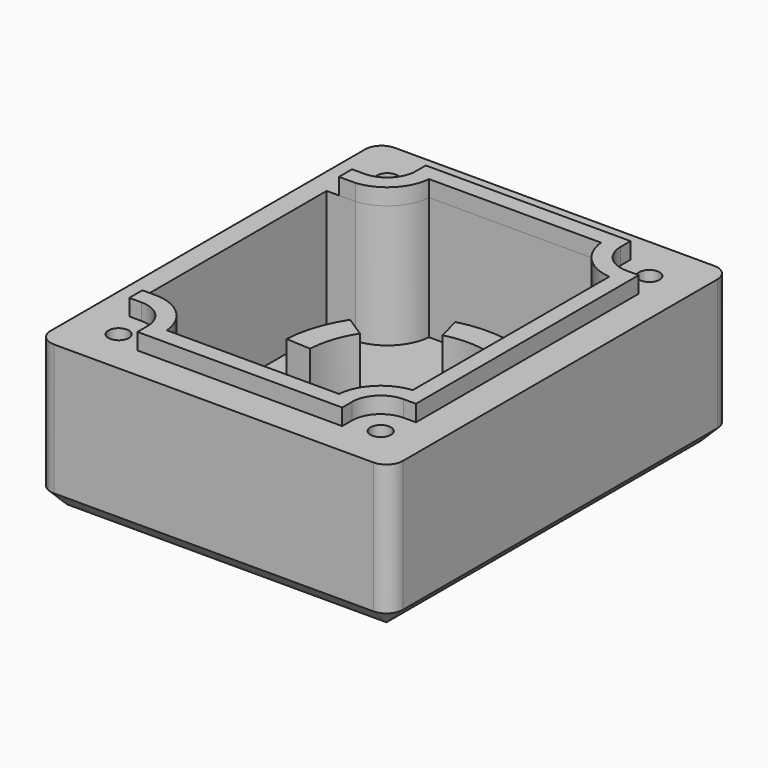
from build123d import *

# Parameters (mm, degrees)
F2_DEPTH  = 2
F3_DEPTH  = 3
F4_R      = 4.5
F5_DEPTH  = 5
F7_D      = 2.5
F8_R      = 4.5
F9_DEPTH  = 2
F10_DEPTH = 10
F11_DEPTH = 5
F12_DEPTH = 5
F13_R     = 4.5
F14_DEPTH = 15
F16_DEPTH = 7
F18_COUNT = 5
F19_SIZE  = 1.99999


# Not quite as in the source:
# - a fillet or chamfer is up to 0.001 mm smaller than in the source, because OpenCascade refuses the exact size


with BuildPart() as f2:
    # F1 (on Top) → F2 (new body)
    with BuildSketch(Plane.XY):
        with BuildLine():
            Line((-15.14, 17), (-16.64, 17))
            Line((-16.64, 17), (-16.64, -17))
            Line((-16.64, -17), (-15.14, -17))
            ThreePointArc((-15.14, -17), (-12.6651262658, -18.0251262658), (-11.64, -20.5))
            Line((-11.64, -20.5), (-11.64, -22))
            Line((-11.64, -22), (13.36, -22))
            Line((13.36, -22), (13.36, -20.5))
            ThreePointArc((13.36, -20.5), (14.3851262658, -18.0251262658), (16.86, -17))
            Line((16.86, -17), (18.36, -17))
            Line((18.36, -17), (18.36, 17))
            Line((18.36, 17), (16.86, 17))
            ThreePointArc((16.86, 17), (14.3851262658, 18.0251262658), (13.36, 20.5))
            Line((13.36, 20.5), (13.36, 22))
            Line((13.36, 22), (-11.64, 22))
            Line((-11.64, 22), (-11.64, 20.5))
            ThreePointArc((-11.64, 20.5), (-12.6651262658, 18.0251262658), (-15.14, 17))
        make_face()
    extrude(amount=F2_DEPTH)

    # F0 (on Top) → F3 (join)
    with BuildSketch(Plane.XY):
        with BuildLine():
            Line((20.36, 26), (-18.64, 26))
            ThreePointArc((-18.64, 26), (-20.0542135624, 25.4142135624), (-20.64, 24))
            Line((-20.64, 24), (-20.64, -24))
            ThreePointArc((-20.64, -24), (-20.0542135624, -25.4142135624), (-18.64, -26))
            Line((-18.64, -26), (20.36, -26))
            ThreePointArc((20.36, -26), (21.7742135624, -25.4142135624), (22.36, -24))
            Line((22.36, -24), (22.36, 24))
            ThreePointArc((22.36, 24), (21.7742135624, 25.4142135624), (20.36, 26))
        make_face()
        with BuildLine():
            Line((-17.64, -18), (-17.64, 18))
            Line((-17.64, 18), (-15.14, 18))
            ThreePointArc((-15.14, 18), (-13.372233047, 18.732233047), (-12.64, 20.5))
            Line((-12.64, 20.5), (-12.64, 23))
            Line((-12.64, 23), (14.36, 23))
            Line((14.36, 23), (14.36, 20.5))
            ThreePointArc((14.36, 20.5), (15.092233047, 18.732233047), (16.86, 18))
            Line((16.86, 18), (19.36, 18))
            Line((19.36, 18), (19.36, -18))
            Line((19.36, -18), (16.86, -18))
            ThreePointArc((16.86, -18), (15.092233047, -18.732233047), (14.36, -20.5))
            Line((14.36, -20.5), (14.36, -23))
            Line((14.36, -23), (-12.64, -23))
            Line((-12.64, -23), (-12.64, -20.5))
            ThreePointArc((-12.64, -20.5), (-13.372233047, -18.732233047), (-15.14, -18))
            Line((-15.14, -18), (-17.64, -18))
        make_face(mode=Mode.SUBTRACT)
        with BuildLine():
            Line((-15.14, 18), (-17.64, 18))
            Line((-17.64, 18), (-17.64, -18))
            Line((-17.64, -18), (-15.14, -18))
            ThreePointArc((-15.14, -18), (-13.372233047, -18.732233047), (-12.64, -20.5))
            Line((-12.64, -20.5), (-12.64, -23))
            Line((-12.64, -23), (14.36, -23))
            Line((14.36, -23), (14.36, -20.5))
            ThreePointArc((14.36, -20.5), (15.092233047, -18.732233047), (16.86, -18))
            Line((16.86, -18), (19.36, -18))
            Line((19.36, -18), (19.36, 18))
            Line((19.36, 18), (16.86, 18))
            ThreePointArc((16.86, 18), (15.092233047, 18.732233047), (14.36, 20.5))
            Line((14.36, 20.5), (14.36, 23))
            Line((14.36, 23), (-12.64, 23))
            Line((-12.64, 23), (-12.64, 20.5))
            ThreePointArc((-12.64, 20.5), (-13.372233047, 18.732233047), (-15.14, 18))
        make_face()
    extrude(amount=-F3_DEPTH)

    # F4 (on face) → F5 (cut, through all)
    with BuildSketch(Plane(origin=(0, 0, -3), x_dir=(1, 0, 0), z_dir=(0, 0, -1))):
        with Locations((2.36, 0)):
            Circle(F4_R)
    extrude(amount=-F5_DEPTH, mode=Mode.SUBTRACT)

    # F7 (through all)
    with Locations(Plane(origin=(0, 0, -3), x_dir=(1, 0, 0), z_dir=(0, 0, -1))):
        with Locations((-15.14, 20.5), (16.86, 20.5), (16.86, -20.5), (-15.14, -20.5)):
            Hole(F7_D / 2)

    # F8 (on face) → F9 (cut, through all)
    with BuildSketch(Plane.XY.offset(2)):
        with BuildLine():
            Line((11.36, 20), (-9.64, 20))
            ThreePointArc((-9.64, 20), (-11.234875162, 16.594875162), (-14.64, 15))
            Line((-14.64, 15), (-16.64, 15))
            Line((-16.64, 15), (-16.64, -15))
            Line((-16.64, -15), (-14.64, -15))
            ThreePointArc((-14.64, -15), (-11.234875162, -16.594875162), (-9.64, -20))
            Line((-9.64, -20), (11.36, -20))
            ThreePointArc((11.36, -20), (12.954875162, -16.594875162), (16.36, -15))
            Line((16.36, -15), (16.36, 15))
            ThreePointArc((16.36, 15), (12.954875162, 16.594875162), (11.36, 20))
        make_face()
        with Locations((2.36, 0)):
            Circle(F8_R, mode=Mode.SUBTRACT)
    extrude(amount=-F9_DEPTH, mode=Mode.SUBTRACT)

    # F10 (add): a face of the model
    f10_faces = [f2.faces().sort_by_distance(p)[0] for p in [
        (0.86, 25.3252407837, -3),
    ]]
    extrude(f10_faces, amount=F10_DEPTH)

    # F11 (add): a face of the model
    f11_faces = [f2.faces().sort_by_distance(p)[0] for p in [
        (0.86, 25.3252407837, 0),
    ]]
    extrude(f11_faces, amount=F11_DEPTH)

    # F12 (add): a face of the model
    f12_faces = [f2.faces().sort_by_distance(p)[0] for p in [
        (12.7977722881, -21.25, 2),
    ]]
    extrude(f12_faces, amount=F12_DEPTH)

    # F13 (on face) → F14 (cut)
    with BuildSketch(Plane.XY.offset(5)):
        with BuildLine():
            Line((-18.14, -15), (-16.64, -15))
            Line((-16.64, -15), (-14.64, -15))
            ThreePointArc((-14.64, -15), (-11.234875162, -16.594875162), (-9.64, -20))
            Line((-9.64, -20), (11.36, -20))
            ThreePointArc((11.36, -20), (12.954875162, -16.594875162), (16.36, -15))
            Line((16.36, -15), (16.36, 15))
            ThreePointArc((16.36, 15), (12.954875162, 16.594875162), (11.36, 20))
            Line((11.36, 20), (-9.64, 20))
            ThreePointArc((-9.64, 20), (-11.234875162, 16.594875162), (-14.64, 15))
            Line((-14.64, 15), (-16.64, 15))
            Line((-16.64, 15), (-18.14, 15))
            Line((-18.14, 15), (-18.14, -15))
        make_face()
        with Locations((2.36, 0)):
            Circle(F13_R, mode=Mode.SUBTRACT)
    extrude(amount=-F14_DEPTH, mode=Mode.SUBTRACT)



with BuildPart() as f16:
    # F15 (on face) → F16 (new body)
    with BuildSketch(Plane.XY.offset(-10)):
        with BuildLine():
            ThreePointArc((-0.4870094961, 10.6251840892), (2.36, 11), (5.2070094961, 10.6251840892))
            Line((5.2070094961, 10.6251840892), (5.9834666315, 13.522961568))
            ThreePointArc((5.9834666315, 13.522961568), (2.36, 14), (-1.2634666314, 13.5229615681))
            Line((-1.2634666314, 13.522961568), (-0.4870094961, 10.6251840892))
        make_face()
    extrude(amount=F16_DEPTH)


with BuildPart() as f2_1:
    add(f2.part)

    add(f16.part)  # F18 merges F16
    # F18: F16 ×5 about axis
    f18_axis = Axis((2.36, 0, 10.6210738979), (0, 0, 1))
    for i in range(1, F18_COUNT):
        add(f16.part.rotate(f18_axis, i * 360 / F18_COUNT))

    # F19 (size 2 in the source; OpenCascade refuses exactly that, so slightly less here)
    f19_edges = [f2_1.edges().sort_by_distance(p)[0] for p in [
        (0.86, -26, -13),
        (-20.64, 0, -13),
        (0.86, 26, -13),
    ]]
    chamfer(f19_edges, length=F19_SIZE)


solid = f2_1.part
